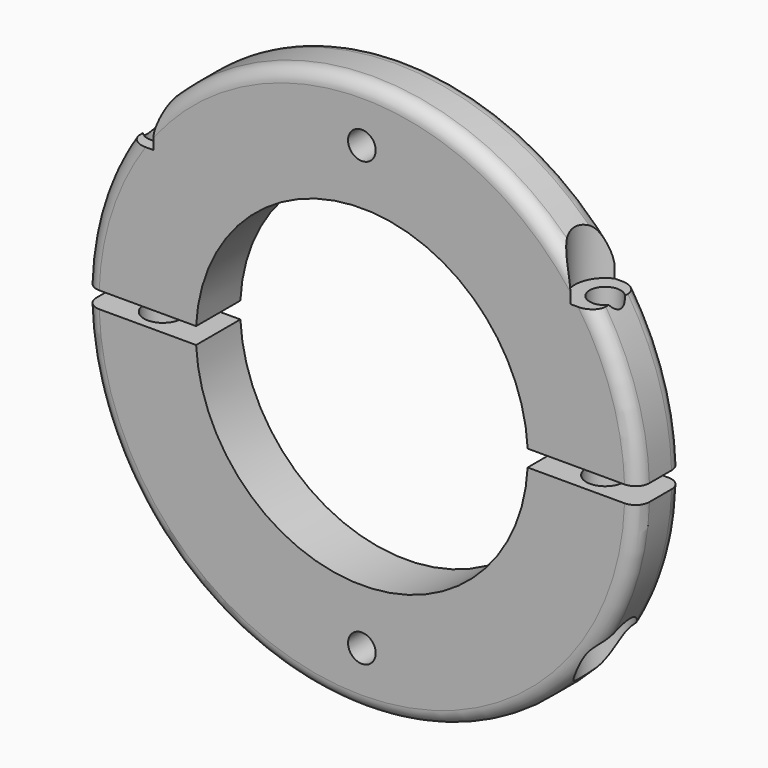
from build123d import *
from build123d import SkipClean  # not in build123d's __all__

# Parameters (mm, degrees)
F1_DEPTH       = 6.35
F4_D           = 8.636
F4_DEPTH       = 38.1
F4_START       = 34.4898158
F4_CBORE_D     = 11.43
F4_CBORE_DEPTH = 5.08
F4_TIP         = 2.594516153
F7_D           = 7.112
F7_DEPTH       = 63.5
F7_CBORE_D     = 13.97
F7_CBORE_DEPTH = 29.21
F7_TIP         = 2.1366603613
F8_T2_ANGLE    = 112.1601252381
F8_T4_ANGLE    = 112.1601252381
F8_T6_ANGLE    = 45.3040515067
F8_T8_ANGLE    = 45.3040515067
F8_T10_ANGLE   = 45.3040515067
F8_T12_ANGLE   = 45.3040515067
F8_2_T2_ANGLE  = 190.8780025379
F8_2_T4_ANGLE  = 190.8780025379
F11_D          = 6.35
F11_DEPTH      = 38.1
F11_START      = 19.05
F11_TIP        = 1.9077324654
F11_2_D        = 6.35
F11_2_DEPTH    = 38.1
F11_2_START    = 19.05
F11_2_TIP      = 1.9077324654


# Not quite as in the source:
# - a fillet or chamfer that OpenCascade refuses, or shapes differently, is made with other operations: its cross-section is extruded or revolved along the edge and cut away or added
# - after a boolean that leaves OpenCascade's solid faulty, fix() repairs it


with BuildPart() as f1:
    # F0 (on Front) → F1 (new body, symmetric)
    with BuildSketch(Plane.XZ):
        with BuildLine():
            ThreePointArc((63.4719124015, 1.8884745421), (0, 63.5), (-63.4719124015, 1.8884745421))
            Line((-63.4719124015, 1.8884745421), (-38.0531689075, 1.8884745421))
            ThreePointArc((-38.0531689075, 1.8884745421), (0, 38.1), (38.0531689075, 1.8884745421))
            Line((38.0531689075, 1.8884745421), (63.4719124015, 1.8884745421))
        make_face()
    extrude(amount=F1_DEPTH, both=True)

    # F7
    with Locations(Plane.XY.offset(63.5)):
        with Locations((50.7719124015, 0), (-50.7719124015, 0)):
            CounterBoreHole(F7_D / 2, F7_CBORE_D / 2, F7_CBORE_DEPTH, depth=F7_DEPTH)
            with Locations((0, 0, -(F7_DEPTH + F7_TIP / 2))):  # 118° drill point
                Cone(0, F7_D / 2, F7_TIP, mode=Mode.SUBTRACT)

    # F8: fillet of radius 3.175 on 6 edges, made by hand

    # F8_s1 → F8_t2 (revolve, cut)
    with BuildSketch(Plane(origin=(0, 0, 0), x_dir=(0, 1, 0), z_dir=(0.558033897, 0, -0.8298181546))):
        with BuildLine():
            ThreePointArc((3.175, 63.5), (5.4200640303, 62.5700640303), (6.35, 60.325))
            Line((6.35, 60.325), (6.35, 63.5))
            Line((6.35, 63.5), (3.175, 63.5))
        make_face()
    revolve(axis=Axis((0, 6.35, 0), (0, -1, 0)), revolution_arc=F8_T2_ANGLE, mode=Mode.SUBTRACT)

    # F8_s3 → F8_t4 (revolve, cut)
    with BuildSketch(Plane(origin=(0, 0, 0), x_dir=(0, 1, 0), z_dir=(0.558033897, 0, -0.8298181546))):
        with BuildLine():
            ThreePointArc((-6.35, 60.325), (-5.4200640303, 62.5700640303), (-3.175, 63.5))
            Line((-3.175, 63.5), (-6.35, 63.5))
            Line((-6.35, 63.5), (-6.35, 60.325))
        make_face()
    revolve(axis=Axis((0, -6.35, 0), (0, -1, 0)), revolution_arc=F8_T4_ANGLE, mode=Mode.SUBTRACT)

    # F8_s5 → F8_t6 (revolve, cut)
    with BuildSketch(Plane(origin=(0, 0, 0), x_dir=(0, 1, 0), z_dir=(0.6407256686, 0, 0.7677698989))):
        with BuildLine():
            ThreePointArc((-6.35, 60.325), (-5.4200640303, 62.5700640303), (-3.175, 63.5))
            Line((-3.175, 63.5), (-6.35, 63.5))
            Line((-6.35, 63.5), (-6.35, 60.325))
        make_face()
    revolve(axis=Axis((0, -6.35, 0), (0, -1, 0)), revolution_arc=F8_T6_ANGLE, mode=Mode.SUBTRACT)

    # F8_s7 → F8_t8 (revolve, cut)
    with BuildSketch(Plane(origin=(0, 0, 0), x_dir=(0, 1, 0), z_dir=(0.6407256686, 0, 0.7677698989))):
        with BuildLine():
            ThreePointArc((3.175, 63.5), (5.4200640303, 62.5700640303), (6.35, 60.325))
            Line((6.35, 60.325), (6.35, 63.5))
            Line((6.35, 63.5), (3.175, 63.5))
        make_face()
    revolve(axis=Axis((0, 6.35, 0), (0, -1, 0)), revolution_arc=F8_T8_ANGLE, mode=Mode.SUBTRACT)

    # F8_s9 → F8_t10 (revolve, cut)
    with BuildSketch(Plane(origin=(0, 0, 0), x_dir=(0, 1, 0), z_dir=(-0.0951177907, 0, -0.9954660245))):
        with BuildLine():
            ThreePointArc((-6.35, 60.325), (-5.4200640303, 62.5700640303), (-3.175, 63.5))
            Line((-3.175, 63.5), (-6.35, 63.5))
            Line((-6.35, 63.5), (-6.35, 60.325))
        make_face()
    revolve(axis=Axis((0, -6.35, 0), (0, -1, 0)), revolution_arc=F8_T10_ANGLE, mode=Mode.SUBTRACT)

    # F8_s11 → F8_t12 (revolve, cut)
    with BuildSketch(Plane(origin=(0, 0, 0), x_dir=(0, 1, 0), z_dir=(-0.0951177907, 0, -0.9954660245))):
        with BuildLine():
            ThreePointArc((6.35, 60.325), (5.4200640303, 62.5700640303), (3.175, 63.5))
            Line((3.175, 63.5), (6.35, 63.5))
            Line((6.35, 63.5), (6.35, 60.325))
        make_face()
    with SkipClean():  # cleaning this boolean's faces spoils the solid; the shape is the same uncleaned
        revolve(axis=Axis((0, 6.35, 0), (0, -1, 0)), revolution_arc=F8_T12_ANGLE, mode=Mode.SUBTRACT)

    # F11
    # its depths count from where the whole tool has entered the part; down to there all is cleared
    with Locations(Plane.XZ.offset(25.4).offset(-F11_START)):
        with Locations((0, 50.8), (0, -50.8)):
            Hole(F11_D / 2, depth=F11_DEPTH)
            with Locations((0, 0, -(F11_DEPTH + F11_TIP / 2))):  # 118° drill point
                Cone(0, F11_D / 2, F11_TIP, mode=Mode.SUBTRACT)

    add(f1.part.fix(), mode=Mode.REPLACE)


with BuildPart() as f1b:
    # F0 (on Front) → F1, piece 2 (new body, symmetric)
    with BuildSketch(Plane.XZ):
        with BuildLine():
            ThreePointArc((38.051514292, -1.9215254579), (0, -38.1), (-38.051514292, -1.9215254579))
            Line((-38.051514292, -1.9215254579), (-63.4709204275, -1.9215254579))
            ThreePointArc((-63.4709204275, -1.9215254579), (0, -63.5), (63.4709204275, -1.9215254579))
            Line((63.4709204275, -1.9215254579), (38.051514292, -1.9215254579))
        make_face()
    extrude(amount=F1_DEPTH, both=True)

    # F4
    # its depths count from where the whole tool has entered the part; down to there all is cleared
    with Locations(Plane(origin=(0, 0, -63.5), x_dir=(1, 0, 0), z_dir=(0, 0, -1)).offset(-F4_START)):
        with Locations((50.7709204275, 0), (-50.7709204275, 0)):
            CounterBoreHole(F4_D / 2, F4_CBORE_D / 2, F4_CBORE_DEPTH, depth=F4_DEPTH)
            with Locations((0, 0, -(F4_DEPTH + F4_TIP / 2))):  # 118° drill point
                Cone(0, F4_D / 2, F4_TIP, mode=Mode.SUBTRACT)

    # F8#2: fillet of radius 3.175 on 2 edges, made by hand

    # F8_2_s1 → F8_2_t2 (revolve, cut)
    with BuildSketch(Plane(origin=(0, 0, 0), x_dir=(0, 1, 0), z_dir=(0.094785971, 0, 0.9954976744))):
        with BuildLine():
            ThreePointArc((-3.175, 63.5), (-5.4200640303, 62.5700640303), (-6.35, 60.325))
            Line((-6.35, 60.325), (-6.35, 63.5))
            Line((-6.35, 63.5), (-3.175, 63.5))
        make_face()
    revolve(axis=Axis((0, -6.35, 0), (0, -1, 0)), revolution_arc=F8_2_T2_ANGLE, mode=Mode.SUBTRACT)

    # F8_2_s3 → F8_2_t4 (revolve, cut)
    with BuildSketch(Plane(origin=(0, 0, 0), x_dir=(0, 1, 0), z_dir=(0.094785971, 0, 0.9954976744))):
        with BuildLine():
            ThreePointArc((3.175, 63.5), (5.4200640303, 62.5700640303), (6.35, 60.325))
            Line((6.35, 60.325), (6.35, 63.5))
            Line((6.35, 63.5), (3.175, 63.5))
        make_face()
    revolve(axis=Axis((0, 6.35, 0), (0, -1, 0)), revolution_arc=F8_2_T4_ANGLE, mode=Mode.SUBTRACT)

    # F11#2
    # its depths count from where the whole tool has entered the part; down to there all is cleared
    with Locations(Plane.XZ.offset(25.4).offset(-F11_2_START)):
        with Locations((0, 50.8), (0, -50.8)):
            Hole(F11_2_D / 2, depth=F11_2_DEPTH)
            with Locations((0, 0, -(F11_2_DEPTH + F11_2_TIP / 2))):  # 118° drill point
                Cone(0, F11_2_D / 2, F11_2_TIP, mode=Mode.SUBTRACT)


solid = Compound([f1.part, f1b.part])
